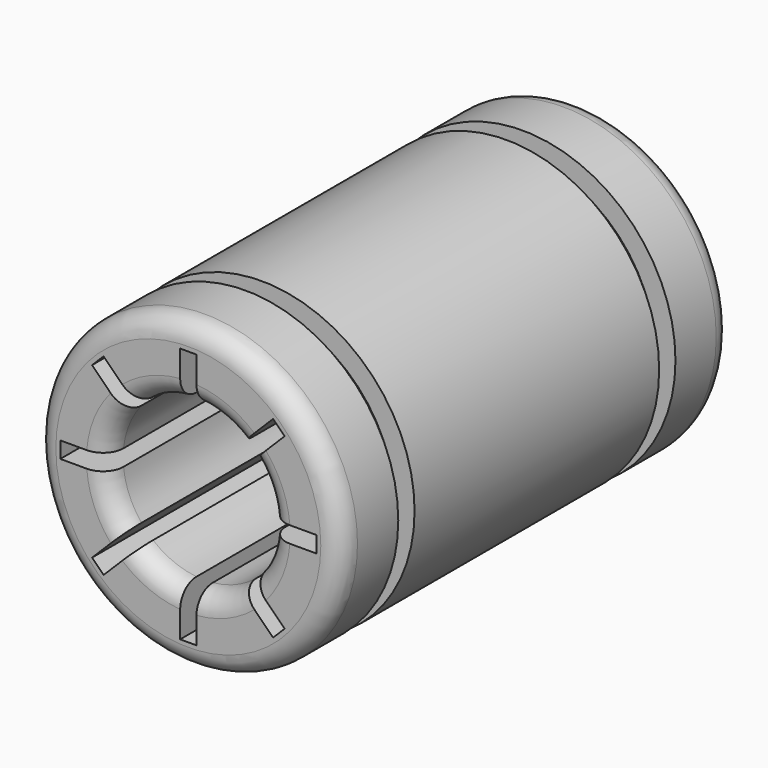
from build123d import *

# Parameters (mm, degrees)
F0_R     = 7.5
F1_DEPTH = 12
F2_R     = 1
F3_W     = 1
F3_H     = 1


# Not quite as in the source:
# - a pattern or mirror of a feature is missing from the dataset's text; its kind, count and spacing are read off the source's solid


with BuildPart() as f1:
    # F0 (on Front) → F1 (new body, symmetric)
    with BuildSketch(Plane.XZ):
        Circle(F0_R)
        with BuildLine():
            ThreePointArc((3.0970921684, 2.5314067434), (3.69551813, 1.5307337295), (3.9799497484, 0.4))
            Line((3.9799497484, 0.4), (6.2799497484, 0.4))
            Line((6.2799497484, 0.4), (6.2799497484, -0.4))
            Line((6.2799497484, -0.4), (3.9799497484, -0.4))
            ThreePointArc((3.9799497484, -0.4), (3.69551813, -1.5307337295), (3.0970921684, -2.5314067434))
            Line((3.0970921684, -2.5314067434), (4.7234377651, -4.1577523401))
            Line((4.7234377651, -4.1577523401), (4.1577523401, -4.7234377651))
            Line((4.1577523401, -4.7234377651), (2.5314067434, -3.0970921684))
            ThreePointArc((2.5314067434, -3.0970921684), (1.5307337295, -3.69551813), (0.4, -3.9799497484))
            Line((0.4, -3.9799497484), (0.4, -6.2799497484))
            Line((0.4, -6.2799497484), (-0.4, -6.2799497484))
            Line((-0.4, -6.2799497484), (-0.4, -3.9799497484))
            ThreePointArc((-0.4, -3.9799497484), (-1.5307337295, -3.69551813), (-2.5314067434, -3.0970921684))
            Line((-2.5314067434, -3.0970921684), (-4.1577523401, -4.7234377651))
            Line((-4.1577523401, -4.7234377651), (-4.7234377651, -4.1577523401))
            Line((-4.7234377651, -4.1577523401), (-3.0970921684, -2.5314067434))
            ThreePointArc((-3.0970921684, -2.5314067434), (-3.69551813, -1.5307337295), (-3.9799497484, -0.4))
            Line((-3.9799497484, -0.4), (-6.2799497484, -0.4))
            Line((-6.2799497484, -0.4), (-6.2799497484, 0.4))
            Line((-6.2799497484, 0.4), (-3.9799497484, 0.4))
            ThreePointArc((-3.9799497484, 0.4), (-3.69551813, 1.5307337295), (-3.0970921684, 2.5314067434))
            Line((-3.0970921684, 2.5314067434), (-4.7234377651, 4.1577523401))
            Line((-4.7234377651, 4.1577523401), (-4.1577523401, 4.7234377651))
            Line((-4.1577523401, 4.7234377651), (-2.5314067434, 3.0970921684))
            ThreePointArc((-2.5314067434, 3.0970921684), (-1.5307337295, 3.69551813), (-0.4, 3.9799497484))
            Line((-0.4, 3.9799497484), (-0.4, 6.2799497484))
            Line((-0.4, 6.2799497484), (0.4, 6.2799497484))
            Line((0.4, 6.2799497484), (0.4, 3.9799497484))
            ThreePointArc((0.4, 3.9799497484), (1.5307337295, 3.69551813), (2.5314067434, 3.0970921684))
            Line((2.5314067434, 3.0970921684), (4.1577523401, 4.7234377651))
            Line((4.1577523401, 4.7234377651), (4.7234377651, 4.1577523401))
            Line((4.7234377651, 4.1577523401), (3.0970921684, 2.5314067434))
        make_face(mode=Mode.SUBTRACT)
    extrude(amount=F1_DEPTH, both=True)

    # F2
    f2_edges = [f1.edges().sort_by_distance(p)[0] for p in [
        (-7.5, -12, 0),
        (-1.530734, -12, 3.695518),
        (-3.695518, -12, 1.530734),
        (-3.695518, -12, -1.530734),
        (-1.530734, -12, -3.695518),
        (1.530734, -12, -3.695518),
        (3.695518, -12, -1.530734),
        (3.695518, -12, 1.530734),
        (1.530734, -12, 3.695518),
        (-7.5, 12, 0),
        (3.695518, 12, -1.530734),
        (3.695518, 12, 1.530734),
        (1.530734, 12, 3.695518),
        (-1.530734, 12, 3.695518),
        (-3.695518, 12, 1.530734),
        (-3.695518, 12, -1.530734),
        (-1.530734, 12, -3.695518),
        (1.530734, 12, -3.695518),
    ]]
    fillet(f2_edges, radius=F2_R)

    # F3 (on Right) → F4 (revolve, cut)
    with BuildSketch(Plane.YZ):
        with Locations((-8, 7)):
            Rectangle(F3_W, F3_H)
    f4 = revolve(axis=Axis((0, 11.2657039426, 0), (0, 1, 0)), mode=Mode.SUBTRACT)

    # F4_copies: F4 across plane
    add(f4.mirror(Plane.ZX), mode=Mode.SUBTRACT)


solid = f1.part
